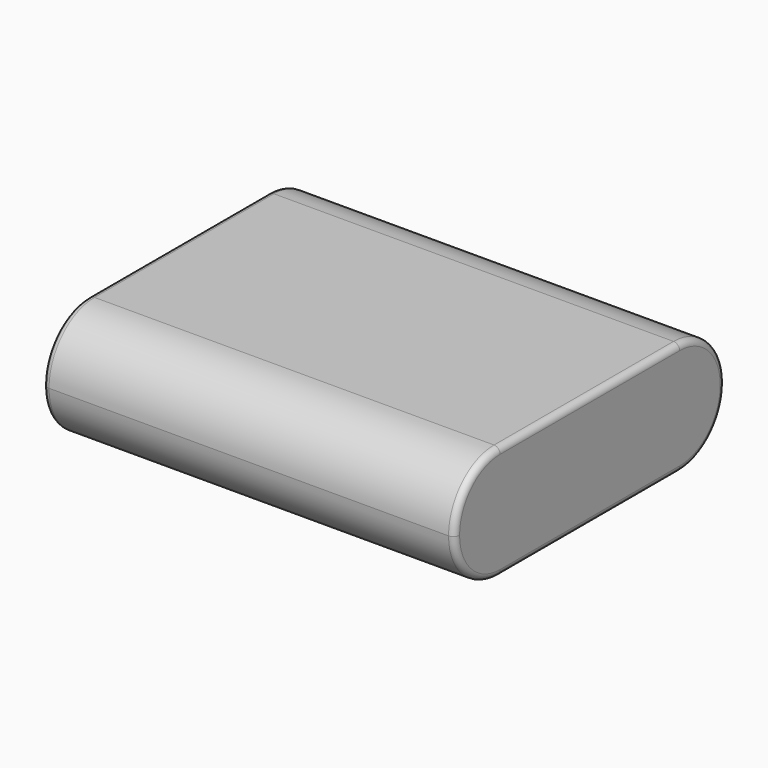
from build123d import *

# Parameters (mm, degrees)
F1_W     = 67
F1_H     = 55
F2_DEPTH = 18.5
F3_R     = 9.24999
F4_R     = 1


# Not quite as in the source:
# - a fillet or chamfer is up to 0.001 mm smaller than in the source, because OpenCascade refuses the exact size


with BuildPart() as f2:
    # F1 (on Top) → F2 (new body)
    with BuildSketch(Plane.XY):
        with Locations((-13.4538196921, -10.3069728613)):
            Rectangle(F1_W, F1_H)
    extrude(amount=F2_DEPTH)

    # F3 (radius 9.25 in the source; OpenCascade refuses exactly that, so slightly less here)
    f3_edges = [f2.edges().sort_by_distance(p)[0] for p in [
        (-13.45382, 17.193027, 18.5),
        (-13.45382, 17.193027, 0),
        (-13.45382, -37.806973, 18.5),
        (-13.45382, -37.806973, 0),
    ]]
    fillet(f3_edges, radius=F3_R)

    # F4
    f4_edges = [f2.edges().sort_by_distance(p)[0] for p in [
        (20.04618, -37.806973, 9.25),
        (20.04618, -35.097714, 2.709259),
        (20.04618, -35.097714, 15.790741),
        (20.04618, -10.306973, 0),
        (20.04618, -10.306973, 18.5),
        (20.04618, 14.483768, 2.709259),
        (20.04618, 14.483768, 15.790741),
        (20.04618, 17.193027, 9.25),
        (-46.95382, 17.193027, 9.25),
        (-46.95382, 14.483768, 2.709259),
        (-46.95382, 14.483768, 15.790741),
        (-46.95382, -10.306973, 0),
        (-46.95382, -10.306973, 18.5),
        (-46.95382, -35.097714, 2.709259),
        (-46.95382, -35.097714, 15.790741),
        (-46.95382, -37.806973, 9.25),
    ]]
    fillet(f4_edges, radius=F4_R)


solid = f2.part
